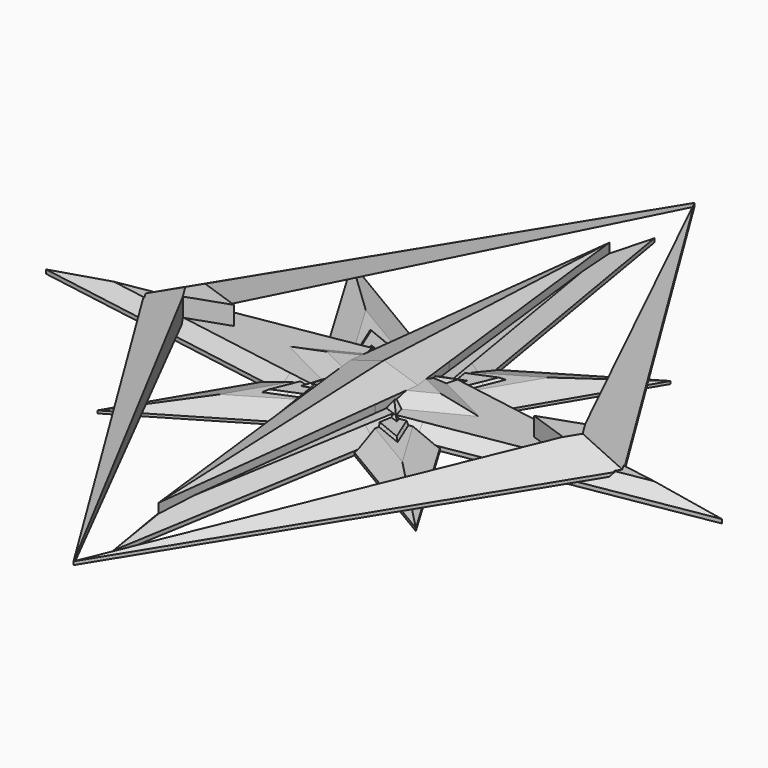
from build123d import *

# Parameters (mm, degrees)
F3_DEPTH      = 2
F4_DEPTH      = 1.033
F5_DEPTH      = 0.8
F6_DEPTH      = 2
F7_DEPTH      = 0.35
F7_DEPTH_BACK = 1
F8_DEPTH      = 0.2
F8_DEPTH_BACK = 1
F9_DEPTH      = 1
F10_T1_DEPTH  = 46.0256343225
F10_T3_DEPTH  = 46.0256343225
F10_T5_DEPTH  = 46.0256343225
F10_T7_DEPTH  = 46.0256343225
F11_T4_DEPTH  = 21.7668274283
F11_T10_DEPTH = 21.7668274283
F11_T17_DEPTH = 21.7668274283
F11_T21_DEPTH = 21.7668274283
F12_T4_DEPTH  = 21.7668274283
F12_T9_DEPTH  = 21.7668274283
F13_T4_DEPTH  = 15.5197526226
F13_T9_DEPTH  = 15.5197526226
F13_T14_DEPTH = 15.9182334476
F13_T19_DEPTH = 15.9182334476
F13_T24_DEPTH = 15.5197526226
F13_T29_DEPTH = 15.5197526226
F13_T34_DEPTH = 15.9182334476
F13_T39_DEPTH = 15.9182334476
F13_T45_DEPTH = 15.5197526226
F13_T49_DEPTH = 15.5197526226
F13_T56_DEPTH = 15.9182334476
F13_T60_DEPTH = 15.9182334476
F13_T67_DEPTH = 15.5197526226
F13_T71_DEPTH = 15.5197526226
F13_T78_DEPTH = 15.9182334476
F13_T82_DEPTH = 15.9182334476
F14_SIZE2     = 3.0922885204
F14_SIZE      = 1.7
F14_2_SIZE2   = 3.0922885204
F14_2_SIZE    = 1.7
F15_SIZE      = 1
F16_SIZE      = 1
F17_SIZE2     = 0.764337492
F17_SIZE      = 2.1


# Not quite as in the source:
# - a fillet or chamfer that OpenCascade refuses, or shapes differently, is made with other operations: its cross-section is extruded or revolved along the edge and cut away or added


with BuildPart() as f3:
    # F0 (on Top) → F3 (new body)
    with BuildSketch(Plane.XY):
        Polygon((-2.9967564624, 25), (0, 25), (0, 28.227372095), (-2.4366995726, 29.0945203591), (-2.51043341, 29.0570785323), align=None)
        Polygon((-2.4366995726, 20.9054796409), (0, 21.772627905), (0, 25), (-2.9967564624, 25), (-2.51043341, 20.9429214677), align=None)
        Polygon((0, 28.227372095), (0, 25), (2.9967564624, 25), (2.51043341, 29.0570785323), (2.4366995726, 29.0945203591), align=None)
        Polygon((0, 25), (0, 21.772627905), (2.4366995726, 20.9054796409), (2.51043341, 20.9429214677), (2.9967564624, 25), align=None)
        Polygon((2.4366995726, 29.0945203591), (2.51043341, 29.0570785323), (2.5031122034, 29.1181546217), align=None)
        Polygon((-2.5031122034, 29.1181546217), (-2.51043341, 29.0570785323), (-2.4366995726, 29.0945203591), align=None)
        Polygon((-2.51043341, 20.9429214677), (-2.5031122034, 20.8818453783), (-2.4366995726, 20.9054796409), align=None)
        Polygon((2.4366995726, 20.9054796409), (2.5031122034, 20.8818453783), (2.51043341, 20.9429214677), align=None)
        Polygon((-2.4366995726, 20.9054796409), (0, 19.6681307291), (0, 21.772627905), align=None)
        Polygon((0, 21.772627905), (0, 19.6681307291), (2.4366995726, 20.9054796409), align=None)
        Polygon((0, 19.6681307291), (0, 0), (2.5031122034, 20.8818453783), (2.4366995726, 20.9054796409), align=None)
        Polygon((-2.5031122034, 20.8818453783), (0, 0), (0, 19.6681307291), (-2.4366995726, 20.9054796409), align=None)
        Polygon((-2.4366995726, 29.0945203591), (0, 30.3318692709), (0, 50), (-2.5031122034, 29.1181546217), align=None)
        Polygon((0, 50), (0, 30.3318692709), (2.4366995726, 29.0945203591), (2.5031122034, 29.1181546217), align=None)
        Polygon((0, 30.3318692709), (0, 28.227372095), (2.4366995726, 29.0945203591), align=None)
        Polygon((-2.4366995726, 29.0945203591), (0, 28.227372095), (0, 30.3318692709), align=None)
    extrude(amount=F3_DEPTH)

    # F0 (on Top) → F4 (join)
    with BuildSketch(Plane.XY):
        Polygon((-3.9748577401, 25), (-2.9967564624, 25), (-2.51043341, 29.0570785323), (-4.7882031367, 27.9004337312), align=None)
        Polygon((-4.7882031367, 22.0995662688), (-2.51043341, 20.9429214677), (-2.9967564624, 25), (-3.9748577401, 25), align=None)
        Polygon((2.51043341, 29.0570785323), (2.9967564624, 25), (3.9748577401, 25), (4.7882031367, 27.9004337312), align=None)
        Polygon((2.9967564624, 25), (2.51043341, 20.9429214677), (4.7882031367, 22.0995662688), (3.9748577401, 25), align=None)
        Polygon((-4.7882031367, 27.9004337312), (-10.5, 25), (-3.9748577401, 25), align=None)
        Polygon((-10.5, 25), (-4.7882031367, 22.0995662688), (-3.9748577401, 25), align=None)
        Polygon((3.9748577401, 25), (10.5, 25), (4.7882031367, 27.9004337312), align=None)
        Polygon((3.9748577401, 25), (4.7882031367, 22.0995662688), (10.5, 25), align=None)
    extrude(amount=F4_DEPTH)

    # F10: chamfer of 2.975 x 0.9666360963 on 4 edges, made by hand

    # F10_s2 → F10_t1 (cut)
    with BuildSketch(Plane(origin=(-4.5589513288, 38.0323808931, 0), x_dir=(0, 0, 1), z_dir=(0.119018229, -0.9928920692, 0))):
        Polygon((1.0333639037, 0), (2, -2.975), (2, 0), align=None)
    extrude(amount=F10_T1_DEPTH, mode=Mode.SUBTRACT)

    # F10_s4 → F10_t3 (cut)
    with BuildSketch(Plane(origin=(-0.9189381567, -7.6661064077, 0), x_dir=(0, 0, 1), z_dir=(0.119018229, 0.9928920692, 0))):
        Polygon((1.0333639037, 0), (2, -2.975), (2, 0), align=None)
    extrude(amount=F10_T3_DEPTH, mode=Mode.SUBTRACT)

    # F10_s6 → F10_t5 (cut)
    with BuildSketch(Plane(origin=(-1.3496614545, 11.2593521653, 0), x_dir=(0, 0, 1), z_dir=(-0.119018229, 0.9928920692, 0))):
        Polygon((2, 2.9759114499), (1.0333639037, 5.9509114499), (2, 5.9509114499), align=None)
    extrude(amount=F10_T5_DEPTH, mode=Mode.SUBTRACT)

    # F10_s8 → F10_t7 (cut)
    with BuildSketch(Plane(origin=(6.8275509401, 56.957839466, 0), x_dir=(0, 0, 1), z_dir=(-0.119018229, -0.9928920692, 0))):
        Polygon((2, 2.9759114499), (1.0333639037, 5.9509114499), (2, 5.9509114499), align=None)
    extrude(amount=F10_T7_DEPTH, mode=Mode.SUBTRACT)

    # F11: chamfer of 1.1 x 2.4706404513 on 2 edges, made by hand


with BuildPart() as f5:
    # F0 (on Top) → F5 (new body)
    with BuildSketch(Plane.XY):
        Polygon((-4.7882031367, 27.9004337312), (-2.51043341, 29.0570785323), (-2.5031122034, 29.1181546217), (-5.4208510121, 30.1564903163), align=None)
        Polygon((-3.9748577401, 25), (-2.9967564624, 25), (-2.51043341, 29.0570785323), (-4.7882031367, 27.9004337312), align=None)
        Polygon((2.51043341, 29.0570785323), (2.9967564624, 25), (3.9748577401, 25), (4.7882031367, 27.9004337312), align=None)
        Polygon((2.5031122034, 29.1181546217), (2.51043341, 29.0570785323), (4.7882031367, 27.9004337312), (5.4208510121, 30.1564903163), align=None)
        Polygon((2.9967564624, 25), (2.51043341, 20.9429214677), (4.7882031367, 22.0995662688), (3.9748577401, 25), align=None)
        Polygon((2.51043341, 20.9429214677), (2.5031122034, 20.8818453783), (5.4208510121, 19.8435096837), (4.7882031367, 22.0995662688), align=None)
        Polygon((-4.7882031367, 22.0995662688), (-2.51043341, 20.9429214677), (-2.9967564624, 25), (-3.9748577401, 25), align=None)
        Polygon((-5.4208510121, 19.8435096837), (-2.5031122034, 20.8818453783), (-2.51043341, 20.9429214677), (-4.7882031367, 22.0995662688), align=None)
        Polygon((-2.4366995726, 20.9054796409), (0, 21.772627905), (0, 25), (-2.9967564624, 25), (-2.51043341, 20.9429214677), align=None)
        Polygon((-2.9967564624, 25), (0, 25), (0, 28.227372095), (-2.4366995726, 29.0945203591), (-2.51043341, 29.0570785323), align=None)
        Polygon((0, 28.227372095), (0, 25), (2.9967564624, 25), (2.51043341, 29.0570785323), (2.4366995726, 29.0945203591), align=None)
        Polygon((0, 25), (0, 21.772627905), (2.4366995726, 20.9054796409), (2.51043341, 20.9429214677), (2.9967564624, 25), align=None)
        Polygon((-2.51043341, 20.9429214677), (-2.5031122034, 20.8818453783), (-2.4366995726, 20.9054796409), align=None)
        Polygon((2.4366995726, 20.9054796409), (2.5031122034, 20.8818453783), (2.51043341, 20.9429214677), align=None)
        Polygon((2.4366995726, 29.0945203591), (2.51043341, 29.0570785323), (2.5031122034, 29.1181546217), align=None)
        Polygon((-2.5031122034, 29.1181546217), (-2.51043341, 29.0570785323), (-2.4366995726, 29.0945203591), align=None)
    extrude(amount=F5_DEPTH)

    # F13: chamfer of 1 x 1.9626105055 on 8 edges, made by hand


with BuildPart() as f6:
    # F0 (on Top) → F6 (new body)
    with BuildSketch(Plane.XY):
        Polygon((-21.2712045759, 25), (0, -9.4556555152), (-16.8706087808, 23.7674756604), (-13.3160147816, 25), (-16.8706087808, 26.2325243396), (0, 59.4556555152), align=None)
    extrude(amount=F6_DEPTH)

    # F14
    f14_edges = [f6.edges().sort_by_distance(p)[0] for p in [
        (-10.635602, 42.227828, 2),
        (-10.635602, 7.772172, 2),
    ]]
    chamfer(f14_edges, length=F14_SIZE, length2=F14_SIZE2)


with BuildPart() as f6b:
    # F0 (on Top) → F6, piece 2 (new body)
    with BuildSketch(Plane.XY):
        Polygon((16.8706087808, 23.7674756604), (0, -9.4556555152), (21.2712045759, 25), (0, 59.4556555152), (16.8706087808, 26.2325243396), (13.3160147816, 25), align=None)
    extrude(amount=F6_DEPTH)

    # F14#2
    f14_2_edges = [f6b.edges().sort_by_distance(p)[0] for p in [
        (10.635602, 7.772172, 2),
        (10.635602, 42.227828, 2),
    ]]
    chamfer(f14_2_edges, length=F14_2_SIZE, length2=F14_2_SIZE2)


with BuildPart() as f7:
    # F1 (on Top) → F7 (new body, two sides)
    with BuildSketch(Plane.XY) as f7_sk:
        Polygon((-6.0690162598, 20.963524832), (-4.4142794795, 25), (-30, 25), align=None)
        Polygon((-30, 25), (-4.4142794795, 25), (-6.0690162598, 29.036475168), align=None)
        Polygon((6.0690162598, 29.036475168), (4.4142794795, 25), (30, 25), align=None)
        Polygon((30, 25), (4.4142794795, 25), (6.0690162598, 20.963524832), align=None)
        Polygon((0, 55), (0, 29.4142794795), (4.036475168, 31.0690162598), align=None)
        Polygon((-4.036475168, 31.0690162598), (0, 29.4142794795), (0, 55), align=None)
        Polygon((0, -5), (0, 0), (0, 20.5857205205), (-4.036475168, 18.9309837402), align=None)
        Polygon((0, 20.5857205205), (0, 0), (0, -5), (4.036475168, 18.9309837402), align=None)
        Polygon((-4.4142794795, 25), (0, 25), (-4.3298268691, 29.3298268691), (-6.0690162598, 29.036475168), align=None)
        Polygon((-4.3298268691, 20.6701731309), (0, 25), (-4.4142794795, 25), (-6.0690162598, 20.963524832), align=None)
        Polygon((-4.036475168, 18.9309837402), (0, 20.5857205205), (0, 25), (-4.3298268691, 20.6701731309), align=None)
        Polygon((0, 25), (0, 20.5857205205), (4.036475168, 18.9309837402), (4.3298268691, 20.6701731309), align=None)
        Polygon((4.4142794795, 25), (0, 25), (4.3298268691, 20.6701731309), (6.0690162598, 20.963524832), align=None)
        Polygon((4.3298268691, 29.3298268691), (0, 25), (4.4142794795, 25), (6.0690162598, 29.036475168), align=None)
        Polygon((0, 29.4142794795), (0, 25), (4.3298268691, 29.3298268691), (4.036475168, 31.0690162598), align=None)
        Polygon((-4.3298268691, 29.3298268691), (0, 25), (0, 29.4142794795), (-4.036475168, 31.0690162598), align=None)
    extrude(amount=F7_DEPTH)
    extrude(f7_sk.sketch, amount=-F7_DEPTH_BACK)

    # F16
    f16_edges = [f7.edges().sort_by_distance(p)[0] for p in [
        (-17.164913, 27.164913, 0.35),
        (-17.164913, 22.835087, 0.35),
        (-2.164913, 7.835087, 0.35),
        (2.164913, 7.835087, 0.35),
        (17.164913, 22.835087, 0.35),
        (17.164913, 27.164913, 0.35),
        (2.164913, 42.164913, 0.35),
        (-2.164913, 42.164913, 0.35),
    ]]
    chamfer(f16_edges, length=F16_SIZE)


with BuildPart() as f8:
    # F1 (on Top) → F8 (new body, two sides)
    with BuildSketch(Plane.XY) as f8_sk:
        Polygon((-6.0690162598, 29.036475168), (-4.3298268691, 29.3298268691), (-7.4811446946, 32.4811446946), align=None)
        Polygon((-7.4811446946, 32.4811446946), (-4.3298268691, 29.3298268691), (-4.036475168, 31.0690162598), align=None)
        Polygon((7.4811446946, 32.4811446946), (4.3298268691, 29.3298268691), (6.0690162598, 29.036475168), align=None)
        Polygon((4.036475168, 31.0690162598), (4.3298268691, 29.3298268691), (7.4811446946, 32.4811446946), align=None)
        Polygon((4.3298268691, 20.6701731309), (4.036475168, 18.9309837402), (7.4811446946, 17.5188553054), align=None)
        Polygon((6.0690162598, 20.963524832), (4.3298268691, 20.6701731309), (7.4811446946, 17.5188553054), align=None)
        Polygon((-7.4811446946, 17.5188553054), (-4.3298268691, 20.6701731309), (-6.0690162598, 20.963524832), align=None)
        Polygon((-7.4811446946, 17.5188553054), (-4.036475168, 18.9309837402), (-4.3298268691, 20.6701731309), align=None)
        Polygon((-4.4142794795, 25), (0, 25), (-4.3298268691, 29.3298268691), (-6.0690162598, 29.036475168), align=None)
        Polygon((-4.3298268691, 29.3298268691), (0, 25), (0, 29.4142794795), (-4.036475168, 31.0690162598), align=None)
        Polygon((0, 29.4142794795), (0, 25), (4.3298268691, 29.3298268691), (4.036475168, 31.0690162598), align=None)
        Polygon((4.3298268691, 29.3298268691), (0, 25), (4.4142794795, 25), (6.0690162598, 29.036475168), align=None)
        Polygon((0, 25), (0, 20.5857205205), (4.036475168, 18.9309837402), (4.3298268691, 20.6701731309), align=None)
        Polygon((4.4142794795, 25), (0, 25), (4.3298268691, 20.6701731309), (6.0690162598, 20.963524832), align=None)
        Polygon((-4.3298268691, 20.6701731309), (0, 25), (-4.4142794795, 25), (-6.0690162598, 20.963524832), align=None)
        Polygon((-4.036475168, 18.9309837402), (0, 20.5857205205), (0, 25), (-4.3298268691, 20.6701731309), align=None)
    extrude(amount=F8_DEPTH)
    extrude(f8_sk.sketch, amount=-F8_DEPTH_BACK)

    # F15
    f15_edges = [f8.edges().sort_by_distance(p)[0] for p in [
        (-5.947712, 28.740572, 0.2),
        (-3.740572, 30.947712, 0.2),
        (3.740572, 30.947712, 0.2),
        (5.947712, 28.740572, 0.2),
        (5.947712, 21.259428, 0.2),
        (3.740572, 19.052288, 0.2),
        (-3.740572, 19.052288, 0.2),
        (-5.947712, 21.259428, 0.2),
    ]]
    chamfer(f15_edges, length=F15_SIZE)


with BuildPart() as f9:
    # F2 (on Top) → F9 (new body)
    with BuildSketch(Plane.XY):
        Polygon((-14.1421356237, 39.1421356237), (0, 25), (14.1421356237, 39.1421356237), (0, 30.724999588), align=None)
        Polygon((-14.1421356237, 10.8578643763), (0, 25), (-14.1421356237, 39.1421356237), (-5.724999588, 25), align=None)
        Polygon((0, 25), (0, 19.275000412), (14.1421356237, 10.8578643763), align=None)
        Polygon((5.724999588, 25), (0, 25), (14.1421356237, 10.8578643763), align=None)
        Polygon((14.1421356237, 39.1421356237), (0, 25), (5.724999588, 25), align=None)
        Polygon((-14.1421356237, 10.8578643763), (0, 19.275000412), (0, 25), align=None)
    extrude(amount=-F9_DEPTH)

    # F17
    f17_edges = [f9.edges().sort_by_distance(p)[0] for p in [
        (7.071068, 34.933568, 0),
        (-7.071068, 34.933568, 0),
        (-9.933568, 32.071068, 0),
        (-9.933568, 17.928932, 0),
        (-7.071068, 15.066432, 0),
        (7.071068, 15.066432, 0),
        (9.933568, 17.928932, 0),
        (9.933568, 32.071068, 0),
    ]]
    f17_side = f9.faces().sort_by_distance((0, 25, 0))[0]
    chamfer(f17_edges, length=F17_SIZE, length2=F17_SIZE2, reference=f17_side)


with BuildPart() as f11_tool2:
    # F11_s3 → F11_t4 (new body)
    with BuildSketch(Plane(origin=(15.4437232982, 7.8422774935, 0), x_dir=(0, 0, 1), z_dir=(-0.8916290603, -0.4527666274, 0))):
        with BuildLine():
            Line((1.0731960001, 24.4838539487), (-0.1071960001, 27.1350577889))
            Line((-0.1071960001, 27.1350577889), (-0.1071960001, 27.1844705979))
            ThreePointArc((-0.1071960001, 27.1844705979), (0.4629019999, 27.0941889034), (1.033, 27.0941889034))
            Line((1.033, 27.0941889034), (1.082412809, 27.0447760944))
            ThreePointArc((1.082412809, 27.0447760944), (1.082412809, 25.7643150215), (1.1226088092, 24.4838539487))
            Line((1.1226088092, 24.4838539487), (1.0731960001, 24.4838539487))
        make_face()
    extrude(amount=F11_T4_DEPTH)

    split(bisect_by=Plane(origin=(-5.9086127834, 0.7082669417, 0), x_dir=(0, 0, 1), z_dir=(-0.9928920692, 0.119018229, 0)), keep=Keep.TOP)

    split(bisect_by=Plane(origin=(7.9400220643, 15.636210762, 0), x_dir=(0, 0, 1), z_dir=(0.4527666274, 0.8916290603, 0)), keep=Keep.TOP)


with BuildPart() as f3_1:
    add(f3.part)

    # F11_t1: cut F11_tool2
    add(f11_tool2.part, mode=Mode.SUBTRACT)


with BuildPart() as f11_tool8:
    # F11_s9 → F11_t10 (new body)
    with BuildSketch(Plane(origin=(-24.1492067118, 12.2628964937, 0), x_dir=(0, 0, 1), z_dir=(0.8916290603, -0.4527666274, 0))):
        with BuildLine():
            Line((-0.1071960001, -17.4463952249), (1.0731960001, -20.0975990651))
            Line((1.0731960001, -20.0975990651), (1.1226088092, -20.0975990651))
            ThreePointArc((1.1226088092, -20.0975990651), (1.082412809, -18.8171379923), (1.082412809, -17.5366769194))
            Line((1.082412809, -17.5366769194), (1.033, -17.4872641103))
            ThreePointArc((1.033, -17.4872641103), (0.4629019999, -17.4872641103), (-0.1071960001, -17.3969824159))
            Line((-0.1071960001, -17.3969824159), (-0.1071960001, -17.4463952249))
        make_face()
    extrude(amount=F11_T10_DEPTH)

    split(bisect_by=Plane(origin=(0, 0, 0), x_dir=(0, 0, 1), z_dir=(-0.9928920692, -0.119018229, 0)), keep=Keep.TOP)

    split(bisect_by=Plane(origin=(-12.2449720606, 24.1139082944, 0), x_dir=(0, 0, 1), z_dir=(0.4527666274, -0.8916290603, 0)), keep=Keep.TOP)


with BuildPart() as f3_2:
    add(f3_1.part)

    # F11_t7: cut F11_tool8
    add(f11_tool8.part, mode=Mode.SUBTRACT)


with BuildPart() as f11_tool15:
    # F11_s16 → F11_t17 (new body)
    with BuildSketch(Plane(origin=(-24.1492067118, 12.2628964937, 0), x_dir=(0, 0, 1), z_dir=(0.8916290603, -0.4527666274, 0))):
        with BuildLine():
            Line((-0.1071960001, -17.4463952249), (1.0731960001, -20.0975990651))
            Line((1.0731960001, -20.0975990651), (1.1226088092, -20.0975990651))
            ThreePointArc((1.1226088092, -20.0975990651), (1.082412809, -18.8171379923), (1.082412809, -17.5366769194))
            Line((1.082412809, -17.5366769194), (1.033, -17.4872641103))
            ThreePointArc((1.033, -17.4872641103), (0.4629019999, -17.4872641103), (-0.1071960001, -17.3969824159))
            Line((-0.1071960001, -17.3969824159), (-0.1071960001, -17.4463952249))
        make_face()
    extrude(amount=F11_T17_DEPTH)

    split(bisect_by=Plane(origin=(-12.2449720606, 24.1139082944, 0), x_dir=(0, 0, 1), z_dir=(-0.4527666274, 0.8916290603, 0)), keep=Keep.TOP)


with BuildPart() as f11_tool19:
    # F11_s20 → F11_t21 (new body)
    with BuildSketch(Plane(origin=(15.4437232982, 7.8422774935, 0), x_dir=(0, 0, 1), z_dir=(-0.8916290603, -0.4527666274, 0))):
        with BuildLine():
            Line((1.0731960001, 24.4838539487), (-0.1071960001, 27.1350577889))
            Line((-0.1071960001, 27.1350577889), (-0.1071960001, 27.1844705979))
            ThreePointArc((-0.1071960001, 27.1844705979), (0.4629019999, 27.0941889034), (1.033, 27.0941889034))
            Line((1.033, 27.0941889034), (1.082412809, 27.0447760944))
            ThreePointArc((1.082412809, 27.0447760944), (1.082412809, 25.7643150215), (1.1226088092, 24.4838539487))
            Line((1.1226088092, 24.4838539487), (1.0731960001, 24.4838539487))
        make_face()
    extrude(amount=F11_T21_DEPTH)

    split(bisect_by=Plane(origin=(7.9400220643, 15.636210762, 0), x_dir=(0, 0, 1), z_dir=(-0.4527666274, -0.8916290603, 0)), keep=Keep.TOP)


with BuildPart() as f11_tool15_1:
    add(f11_tool15.part)

    # F11_t23: intersect F11_tool19
    add(f11_tool19.part, mode=Mode.INTERSECT)


with BuildPart() as f3_3:
    add(f3_2.part)

    # F11_t13: cut F11_tool15
    add(f11_tool15_1.part, mode=Mode.SUBTRACT)

    # F12: chamfer of 1.1 x 2.4706404513 on 2 edges, made by hand


with BuildPart() as f12_tool2:
    # F12_s3 → F12_t4 (new body)
    with BuildSketch(Plane(origin=(3.9642125869, -2.0130155501, 0), x_dir=(0, 0, 1), z_dir=(-0.8916290603, 0.4527666274, 0))):
        Polygon((1.033, 24.5741356431), (-0.067, 27.0447760944), (1.033, 27.0447760944), align=None)
    extrude(amount=F12_T4_DEPTH)

    split(bisect_by=Plane(origin=(5.9086127834, 0.7082669417, 0), x_dir=(0, 0, 1), z_dir=(0.9928920692, 0.119018229, 0)), keep=Keep.TOP)


with BuildPart() as f3_4:
    add(f3_3.part)

    # F12_t1: cut F12_tool2
    add(f12_tool2.part, mode=Mode.SUBTRACT)


with BuildPart() as f12_tool7:
    # F12_s8 → F12_t9 (new body)
    with BuildSketch(Plane(origin=(4.7412708267, 2.4076034501, 0), x_dir=(0, 0, 1), z_dir=(0.8916290603, 0.4527666274, 0))):
        Polygon((1.033, -20.0073173707), (-0.067, -17.5366769194), (1.033, -17.5366769194), align=None)
    extrude(amount=F12_T9_DEPTH)

    split(bisect_by=Plane(origin=(0, 0, 0), x_dir=(0, 0, 1), z_dir=(0.9928920692, -0.119018229, 0)), keep=Keep.TOP)


with BuildPart() as f3_5:
    add(f3_4.part)

    # F12_t6: cut F12_tool7
    add(f12_tool7.part, mode=Mode.SUBTRACT)


with BuildPart() as f13_tool2:
    # F13_s3 → F13_t4 (new body)
    with BuildSketch(Plane(origin=(-9.6074519199, 34.2606938407, 0), x_dir=(0, 0, 1), z_dir=(0.2700066815, -0.9628584485, 0))):
        Polygon((-0.2, -2.9229416808), (0.8, -4.8855521863), (0.8, -2.9229416808), align=None)
    extrude(amount=F13_T4_DEPTH)

    split(bisect_by=Plane(origin=(-10.1845316307, 2.8559666194, 0), x_dir=(0, 0, 1), z_dir=(-0.9628584485, 0.2700066815, 0)), keep=Keep.TOP)


with BuildPart() as f5_1:
    add(f5.part)

    # F13_t1: cut F13_tool2
    add(f13_tool2.part, mode=Mode.SUBTRACT)


with BuildPart() as f13_tool7:
    # F13_s8 → F13_t9 (new body)
    with BuildSketch(Plane(origin=(7.5818957063, 27.0374506884, 0), x_dir=(0, 0, 1), z_dir=(-0.2700066815, -0.9628584485, 0))):
        Polygon((-0.2, 10.5773923945), (0.8, 8.614781889), (0.8, 10.5773923945), align=None)
    extrude(amount=F13_T9_DEPTH)

    split(bisect_by=Plane(origin=(2.814379092, 0.7892137835, 0), x_dir=(0, 0, 1), z_dir=(-0.9628584485, -0.2700066815, 0)), keep=Keep.TOP)


with BuildPart() as f5_2:
    add(f5_1.part)

    # F13_t6: cut F13_tool7
    add(f13_tool7.part, mode=Mode.SUBTRACT)


with BuildPart() as f13_tool12:
    # F13_s13 → F13_t14 (new body)
    with BuildSketch(Plane(origin=(-3.3316132093, -1.1856211754, 0), x_dir=(0, 0, 1), z_dir=(0.9421211452, 0.335272647, 0))):
        Polygon((-0.2, -20.5124531352), (0.8, -22.4750636407), (0.8, -20.5124531352), align=None)
    extrude(amount=F13_T14_DEPTH)

    split(bisect_by=Plane(origin=(6.8772644591, 19.3252158379, 0), x_dir=(0, 0, 1), z_dir=(-0.335272647, -0.9421211452, 0)), keep=Keep.TOP)


with BuildPart() as f5_3:
    add(f5_2.part)

    # F13_t11: cut F13_tool12
    add(f13_tool12.part, mode=Mode.SUBTRACT)


with BuildPart() as f13_tool17:
    # F13_s18 → F13_t19 (new body)
    with BuildSketch(Plane(origin=(-11.6652911154, 4.1513270882, 0), x_dir=(0, 0, 1), z_dir=(0.9421211452, -0.335272647, 0))):
        Polygon((-0.2, -20.5124531352), (0.8, -22.4750636407), (0.8, -20.5124531352), align=None)
    extrude(amount=F13_T19_DEPTH)

    split(bisect_by=Plane(origin=(-6.8772644591, 19.3252158379, 0), x_dir=(0, 0, 1), z_dir=(0.335272647, -0.9421211452, 0)), keep=Keep.TOP)


with BuildPart() as f5_4:
    add(f5_3.part)

    # F13_t16: cut F13_tool17
    add(f13_tool17.part, mode=Mode.SUBTRACT)


with BuildPart() as f13_tool22:
    # F13_s23 → F13_t24 (new body)
    with BuildSketch(Plane(origin=(-3.3914588028, 12.0941257564, 0), x_dir=(0, 0, 1), z_dir=(-0.2700066815, 0.9628584485, 0))):
        Polygon((-0.2, 10.5773923945), (0.8, 8.614781889), (0.8, 10.5773923945), align=None)
    extrude(amount=F13_T24_DEPTH)

    split(bisect_by=Plane(origin=(-2.814379092, 0.7892137835, 0), x_dir=(0, 0, 1), z_dir=(0.9628584485, -0.2700066815, 0)), keep=Keep.TOP)


with BuildPart() as f5_5:
    add(f5_4.part)

    # F13_t21: cut F13_tool22
    add(f13_tool22.part, mode=Mode.SUBTRACT)


with BuildPart() as f13_tool27:
    # F13_s28 → F13_t29 (new body)
    with BuildSketch(Plane(origin=(5.4170150164, 19.3173689087, 0), x_dir=(0, 0, 1), z_dir=(0.2700066815, 0.9628584485, 0))):
        Polygon((-0.2, -2.9229416808), (0.8, -4.8855521863), (0.8, -2.9229416808), align=None)
    extrude(amount=F13_T29_DEPTH)

    split(bisect_by=Plane(origin=(10.1845316307, 2.8559666194, 0), x_dir=(0, 0, 1), z_dir=(0.9628584485, 0.2700066815, 0)), keep=Keep.TOP)


with BuildPart() as f5_6:
    add(f5_5.part)

    # F13_t26: cut F13_tool27
    add(f13_tool27.part, mode=Mode.SUBTRACT)


with BuildPart() as f13_tool32:
    # F13_s33 → F13_t34 (new body)
    with BuildSketch(Plane(origin=(19.1249857161, 6.8060085667, 0), x_dir=(0, 0, 1), z_dir=(-0.9421211452, -0.335272647, 0))):
        Polygon((-0.2, 26.5936041232), (0.8, 24.6309936177), (0.8, 26.5936041232), align=None)
    extrude(amount=F13_T34_DEPTH)

    split(bisect_by=Plane(origin=(8.9161080477, 25.0543967707, 0), x_dir=(0, 0, 1), z_dir=(0.335272647, 0.9421211452, 0)), keep=Keep.TOP)


with BuildPart() as f5_7:
    add(f5_6.part)

    # F13_t31: cut F13_tool32
    add(f13_tool32.part, mode=Mode.SUBTRACT)


with BuildPart() as f13_tool37:
    # F13_s38 → F13_t39 (new body)
    with BuildSketch(Plane(origin=(-4.1280813914, 1.4690603032, 0), x_dir=(0, 0, 1), z_dir=(-0.9421211452, 0.335272647, 0))):
        Polygon((-0.2, 26.5936041232), (0.8, 24.6309936177), (0.8, 26.5936041232), align=None)
    extrude(amount=F13_T39_DEPTH)

    split(bisect_by=Plane(origin=(-8.9161080477, 25.0543967707, 0), x_dir=(0, 0, 1), z_dir=(-0.335272647, 0.9421211452, 0)), keep=Keep.TOP)


with BuildPart() as f5_8:
    add(f5_7.part)

    # F13_t36: cut F13_tool37
    add(f13_tool37.part, mode=Mode.SUBTRACT)


with BuildPart() as f13_tool43:
    # F13_s44 → F13_t45 (new body)
    with BuildSketch(Plane(origin=(-9.6074519199, 34.2606938407, 0), x_dir=(0, 0, 1), z_dir=(0.2700066815, -0.9628584485, 0))):
        Polygon((-0.2, -2.9229416808), (0.8, -4.8855521863), (0.8, -2.9229416808), align=None)
    extrude(amount=F13_T45_DEPTH)

    split(bisect_by=Plane(origin=(-10.1845316307, 2.8559666194, 0), x_dir=(0, 0, 1), z_dir=(0.9628584485, -0.2700066815, 0)), keep=Keep.TOP)


with BuildPart() as f13_tool47:
    # F13_s48 → F13_t49 (new body)
    with BuildSketch(Plane(origin=(7.5818957063, 27.0374506884, 0), x_dir=(0, 0, 1), z_dir=(-0.2700066815, -0.9628584485, 0))):
        Polygon((-0.2, 10.5773923945), (0.8, 8.614781889), (0.8, 10.5773923945), align=None)
    extrude(amount=F13_T49_DEPTH)

    split(bisect_by=Plane(origin=(2.814379092, 0.7892137835, 0), x_dir=(0, 0, 1), z_dir=(0.9628584485, 0.2700066815, 0)), keep=Keep.TOP)


with BuildPart() as f13_tool43_1:
    add(f13_tool43.part)

    # F13_t51: intersect F13_tool47
    add(f13_tool47.part, mode=Mode.INTERSECT)


with BuildPart() as f5_9:
    add(f5_8.part)

    # F13_t41: cut F13_tool43
    add(f13_tool43_1.part, mode=Mode.SUBTRACT)


with BuildPart() as f13_tool54:
    # F13_s55 → F13_t56 (new body)
    with BuildSketch(Plane(origin=(-3.3316132093, -1.1856211754, 0), x_dir=(0, 0, 1), z_dir=(0.9421211452, 0.335272647, 0))):
        Polygon((-0.2, -20.5124531352), (0.8, -22.4750636407), (0.8, -20.5124531352), align=None)
    extrude(amount=F13_T56_DEPTH)

    split(bisect_by=Plane(origin=(6.8772644591, 19.3252158379, 0), x_dir=(0, 0, 1), z_dir=(0.335272647, 0.9421211452, 0)), keep=Keep.TOP)


with BuildPart() as f13_tool58:
    # F13_s59 → F13_t60 (new body)
    with BuildSketch(Plane(origin=(-11.6652911154, 4.1513270882, 0), x_dir=(0, 0, 1), z_dir=(0.9421211452, -0.335272647, 0))):
        Polygon((-0.2, -20.5124531352), (0.8, -22.4750636407), (0.8, -20.5124531352), align=None)
    extrude(amount=F13_T60_DEPTH)

    split(bisect_by=Plane(origin=(-6.8772644591, 19.3252158379, 0), x_dir=(0, 0, 1), z_dir=(-0.335272647, 0.9421211452, 0)), keep=Keep.TOP)


with BuildPart() as f13_tool54_1:
    add(f13_tool54.part)

    # F13_t62: intersect F13_tool58
    add(f13_tool58.part, mode=Mode.INTERSECT)


with BuildPart() as f5_10:
    add(f5_9.part)

    # F13_t52: cut F13_tool54
    add(f13_tool54_1.part, mode=Mode.SUBTRACT)


with BuildPart() as f13_tool65:
    # F13_s66 → F13_t67 (new body)
    with BuildSketch(Plane(origin=(-3.3914588028, 12.0941257564, 0), x_dir=(0, 0, 1), z_dir=(-0.2700066815, 0.9628584485, 0))):
        Polygon((-0.2, 10.5773923945), (0.8, 8.614781889), (0.8, 10.5773923945), align=None)
    extrude(amount=F13_T67_DEPTH)

    split(bisect_by=Plane(origin=(-2.814379092, 0.7892137835, 0), x_dir=(0, 0, 1), z_dir=(-0.9628584485, 0.2700066815, 0)), keep=Keep.TOP)


with BuildPart() as f13_tool69:
    # F13_s70 → F13_t71 (new body)
    with BuildSketch(Plane(origin=(5.4170150164, 19.3173689087, 0), x_dir=(0, 0, 1), z_dir=(0.2700066815, 0.9628584485, 0))):
        Polygon((-0.2, -2.9229416808), (0.8, -4.8855521863), (0.8, -2.9229416808), align=None)
    extrude(amount=F13_T71_DEPTH)

    split(bisect_by=Plane(origin=(10.1845316307, 2.8559666194, 0), x_dir=(0, 0, 1), z_dir=(-0.9628584485, -0.2700066815, 0)), keep=Keep.TOP)


with BuildPart() as f13_tool65_1:
    add(f13_tool65.part)

    # F13_t73: intersect F13_tool69
    add(f13_tool69.part, mode=Mode.INTERSECT)


with BuildPart() as f5_11:
    add(f5_10.part)

    # F13_t63: cut F13_tool65
    add(f13_tool65_1.part, mode=Mode.SUBTRACT)


with BuildPart() as f13_tool76:
    # F13_s77 → F13_t78 (new body)
    with BuildSketch(Plane(origin=(19.1249857161, 6.8060085667, 0), x_dir=(0, 0, 1), z_dir=(-0.9421211452, -0.335272647, 0))):
        Polygon((-0.2, 26.5936041232), (0.8, 24.6309936177), (0.8, 26.5936041232), align=None)
    extrude(amount=F13_T78_DEPTH)

    split(bisect_by=Plane(origin=(8.9161080477, 25.0543967707, 0), x_dir=(0, 0, 1), z_dir=(-0.335272647, -0.9421211452, 0)), keep=Keep.TOP)


with BuildPart() as f13_tool80:
    # F13_s81 → F13_t82 (new body)
    with BuildSketch(Plane(origin=(-4.1280813914, 1.4690603032, 0), x_dir=(0, 0, 1), z_dir=(-0.9421211452, 0.335272647, 0))):
        Polygon((-0.2, 26.5936041232), (0.8, 24.6309936177), (0.8, 26.5936041232), align=None)
    extrude(amount=F13_T82_DEPTH)

    split(bisect_by=Plane(origin=(-8.9161080477, 25.0543967707, 0), x_dir=(0, 0, 1), z_dir=(0.335272647, -0.9421211452, 0)), keep=Keep.TOP)


with BuildPart() as f13_tool76_1:
    add(f13_tool76.part)

    # F13_t84: intersect F13_tool80
    add(f13_tool80.part, mode=Mode.INTERSECT)


with BuildPart() as f5_12:
    add(f5_11.part)

    # F13_t74: cut F13_tool76
    add(f13_tool76_1.part, mode=Mode.SUBTRACT)


solid = Compound([f6.part, f6b.part, f7.part, f8.part, f9.part, f3_5.part, f5_12.part])
